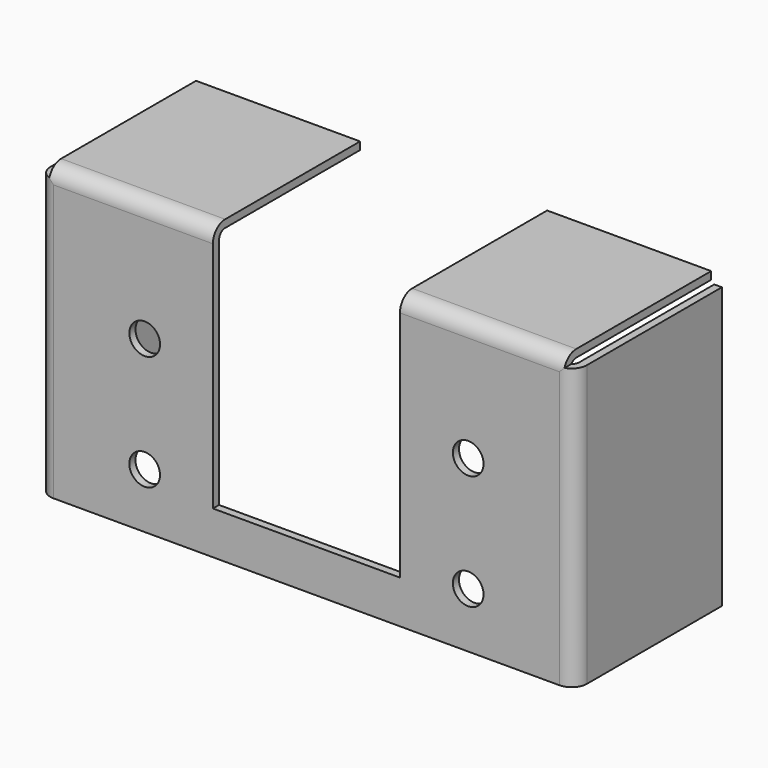
from build123d import *

# Parameters (mm, degrees)
F0_W         = 175
F0_H         = 60
F1_DEPTH     = 95
F3_T         = -2.5
F2_W         = 61
F2_H         = 81
F4_DEPTH     = 60.001
F6_D         = 10
F7_W         = 3.5
F7_H         = 3.5
F8_DEPTH     = 60.001
F9_T1_DEPTH  = 116.5
F9_T3_DEPTH  = 78.5
F9_T5_DEPTH  = 78.5
F10_R        = 2.5
F11_T4_DEPTH = 96.25
F12_R        = 2.5
F13_T4_DEPTH = 96.25


# Not quite as in the source:
# - a fillet or chamfer that OpenCascade refuses, or shapes differently, is made with other operations: its cross-section is extruded or revolved along the edge and cut away or added


with BuildPart() as f1:
    # F0 (on Top) → F1 (new body)
    with BuildSketch(Plane.XY):
        Rectangle(F0_W, F0_H)
    extrude(amount=F1_DEPTH)

    # F3
    f3_openings = [f1.faces().sort_by_distance(p)[0] for p in [
        (0, 30, 47.5),
        (0, 0, 0),
    ]]
    offset(amount=F3_T, openings=f3_openings)

    # F2 (on face) → F4 (cut, through all)
    with BuildSketch(Plane.XZ.offset(30)):
        with Locations((0, 54.5)):
            Rectangle(F2_W, F2_H)
    extrude(amount=-F4_DEPTH, mode=Mode.SUBTRACT)

    # F6 (through all)
    with Locations(Plane.XZ.offset(30)):
        with Locations((52.75, 55.5), (52.75, 18), (-52.75, 18), (-52.75, 55.5)):
            Hole(F6_D / 2)

    # F7 (on face) → F8 (cut, through all)
    with BuildSketch(Plane.XZ.offset(30)):
        with Locations((-85.75, 93.25)):
            Rectangle(F7_W, F7_H)
        with Locations((85.75, 93.25)):
            Rectangle(F7_W, F7_H)
    extrude(amount=-F8_DEPTH, mode=Mode.SUBTRACT)

    # F9: fillet of radius 5 on 4 edges, made by hand

    # F9_s2 → F9_t1 (cut)
    with BuildSketch(Plane.XY.offset(-12.5)):
        with BuildLine():
            ThreePointArc((-87.5, -25), (-86.0355339059, -28.5355339059), (-82.5, -30))
            Line((-82.5, -30), (-87.5, -30))
            Line((-87.5, -30), (-87.5, -25))
        make_face()
        with BuildLine():
            ThreePointArc((82.5, -30), (86.0355339059, -28.5355339059), (87.5, -25))
            Line((87.5, -25), (87.5, -30))
            Line((87.5, -30), (82.5, -30))
        make_face()
    extrude(amount=F9_T1_DEPTH, mode=Mode.SUBTRACT)

    # F9_s4 → F9_t3 (cut)
    with BuildSketch(Plane.YZ.offset(-96.5)):
        with BuildLine():
            ThreePointArc((-30, 90), (-28.5355339059, 93.5355339059), (-25, 95))
            Line((-25, 95), (-30, 95))
            Line((-30, 95), (-30, 90))
        make_face()
    extrude(amount=F9_T3_DEPTH, mode=Mode.SUBTRACT)

    # F9_s6 → F9_t5 (cut)
    with BuildSketch(Plane.YZ.offset(18)):
        with BuildLine():
            ThreePointArc((-30, 90), (-28.5355339059, 93.5355339059), (-25, 95))
            Line((-25, 95), (-30, 95))
            Line((-30, 95), (-30, 90))
        make_face()
    extrude(amount=F9_T5_DEPTH, mode=Mode.SUBTRACT)

    # F10
    f10_edges = [f1.edges().sort_by_distance(p)[0] for p in [
        (57.25, -27.5, 92.5),
    ]]
    fillet(f10_edges, radius=F10_R)

    # F11: fillet of radius 2.5 on 1 edges, made by hand


with BuildPart() as f11_tool2:
    # F11_s3 → F11_t4 (new body)
    with BuildSketch(Plane.XY.offset(96.25)):
        with BuildLine():
            ThreePointArc((82.5, -27.5), (84.267766953, -26.767766953), (85, -25))
            Line((85, -25), (85, -27.5))
            Line((85, -27.5), (82.5, -27.5))
        make_face()
    extrude(amount=-F11_T4_DEPTH)

    split(bisect_by=Plane.XY.offset(91.5), keep=Keep.BOTTOM)


with BuildPart() as f1_1:
    add(f1.part)

    # F11_t1: union F11_tool2
    add(f11_tool2.part)

    # F12
    f12_edges = [f1_1.edges().sort_by_distance(p)[0] for p in [
        (-57.25, -27.5, 92.5),
    ]]
    fillet(f12_edges, radius=F12_R)

    # F13: fillet of radius 2.5 on 1 edges, made by hand


with BuildPart() as f13_tool2:
    # F13_s3 → F13_t4 (new body)
    with BuildSketch(Plane.XY):
        with BuildLine():
            ThreePointArc((-82.5, -27.5), (-84.267766953, -26.767766953), (-85, -25))
            Line((-85, -25), (-85, -27.5))
            Line((-85, -27.5), (-82.5, -27.5))
        make_face()
    extrude(amount=F13_T4_DEPTH)

    split(bisect_by=Plane.XY.offset(91.5), keep=Keep.BOTTOM)


with BuildPart() as f1_2:
    add(f1_1.part)

    # F13_t1: union F13_tool2
    add(f13_tool2.part)


solid = f1_2.part
